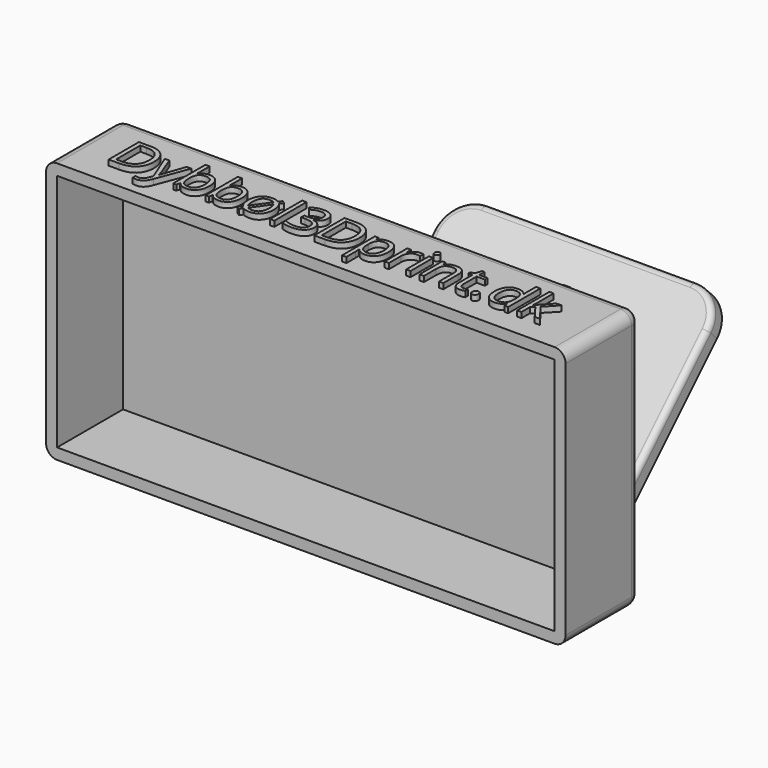
from build123d import *

# Parameters (mm, degrees)
F0_W          = 94.5
F0_H          = 47.5
F1_DEPTH      = 17
F2_T          = -2
F4_DEPTH      = 25
F6_DEPTH      = 1.5
F7_R          = 3
F8_R          = 6
F9_R          = 2
F10_R         = 2
F11_R         = 1
F12_W         = 5
F12_H         = 18
F13_DEPTH     = 51.4984746831
F14_R         = 1
F17_DEPTH     = 8
F18_R         = 1
F19_R         = 1.5
F20_TEXT_SIZE = 9.6209857752
F21_DEPTH     = 1


# Not quite as in the source:
# - Text() gives the source's letters only with a copy of the font that has no kerning and outlines rounded to 1/6400 em; it was checked with that copy


with BuildPart() as f1:
    # F0 (on Front) → F1 (new body)
    with BuildSketch(Plane.XZ):
        Rectangle(F0_W, F0_H)
    extrude(amount=F1_DEPTH)

    # F2
    f2_openings = [f1.faces().sort_by_distance(p)[0] for p in [
        (0, -17, 0),
    ]]
    offset(amount=F2_T, openings=f2_openings)

    # F3 (on Right) → F4 (join, symmetric)
    with BuildSketch(Plane.YZ):
        Polygon((0, 0), (0, -23.75), (14.1421356237, -37.8921356237), (49.4974746831, -2.5367965644), (47.3761543395, -0.4154762208), (14.1421356237, -33.6494949366), (3, -22.5073593129), (3, 13.25), (0, 16.25), align=None)
    extrude(amount=F4_DEPTH, both=True)

    # F5 (on Right) → F6 (join, symmetric)
    with BuildSketch(Plane.YZ):
        Polygon((3, -22.5073593129), (14.1421356237, -33.6494949366), (42.4264068712, -5.3652236891), (3, 7.4926406871), align=None)
    extrude(amount=F6_DEPTH, both=True)

    # F7
    f7_edges = [f1.edges().sort_by_distance(p)[0] for p in [
        (13.25, 14.142136, -33.649495),
        (13.25, 3, -22.507359),
        (-13.25, 14.142136, -33.649495),
        (-13.25, 3, -22.507359),
    ]]
    fillet(f7_edges, radius=F7_R)

    # F8
    f8_edges = [f1.edges().sort_by_distance(p)[0] for p in [
        (0, 14.142136, -37.892136),
        (25, 48.436815, -1.476136),
        (-25, 48.436815, -1.476136),
    ]]
    fillet(f8_edges, radius=F8_R)

    # F9
    f9_edges = [f1.edges().sort_by_distance(p)[0] for p in [
        (-47.25, -8.5, 23.75),
        (-47.25, -8.5, -23.75),
        (47.25, -8.5, -23.75),
        (47.25, -8.5, 23.75),
    ]]
    fillet(f9_edges, radius=F9_R)

    # F10
    f10_edges = [f1.edges().sort_by_distance(p)[0] for p in [
        (0, 0, 23.75),
    ]]
    fillet(f10_edges, radius=F10_R)

    # F11
    f11_edges = [f1.edges().sort_by_distance(p)[0] for p in [
        (1.5, 22.713203, 1.063708),
        (-1.5, 22.713203, 1.063708),
        (25, 29.698485, -18.093146),
        (0, 3, 13.25),
    ]]
    fillet(f11_edges, radius=F11_R)

    # F12 (on face) → F13 (cut, through all)
    with BuildSketch(Plane.XZ.offset(2)):
        with Locations((40.75, 0)):
            Rectangle(F12_W, F12_H)
    extrude(amount=-F13_DEPTH, mode=Mode.SUBTRACT)

    # F14
    f14_edges = [f1.edges().sort_by_distance(p)[0] for p in [
        (43.25, -1, -9),
        (38.25, -1, -9),
        (43.25, -1, 9),
        (38.25, -1, 9),
    ]]
    fillet(f14_edges, radius=F14_R)

    # F16 (on offset) → F17 (join)
    with BuildSketch(Plane(origin=(0, -1.2683982822, -1.2683982822), x_dir=(-1, 0, 0), z_dir=(0, 0.7071067812, 0.7071067812))):
        Polygon((-9.5, -30.7937860532), (-1.5, -30.7937860532), (-1.5, -29.2937860532), (-11, -29.2937860532), (-11, -31.9937860532), (-9.5, -31.9937860532), align=None)
    extrude(amount=F17_DEPTH)

    # F18
    f18_edges = [f1.edges().sort_by_distance(p)[0] for p in [
        (1.5, 23.334524, -20.214466),
        (1.5, 22.273864, -19.153806),
        (9.5, 23.334524, -20.214466),
        (11, 24.183052, -21.062994),
    ]]
    fillet(f18_edges, radius=F18_R)

    # F19
    f19_edges = [f1.edges().sort_by_distance(p)[0] for p in [
        (11, 22.273864, -19.153806),
    ]]
    fillet(f19_edges, radius=F19_R)

    # F20 (on face) → F21 (join)
    with BuildSketch(Plane.XY.offset(23.75)):
        with Locations((-40, -13)):
            Text('Dybbøl3Dprint.dk', F20_TEXT_SIZE, font='Open Sans', text_align=(TextAlign.LEFT, TextAlign.BOTTOM))
    extrude(amount=F21_DEPTH)


solid = f1.part
